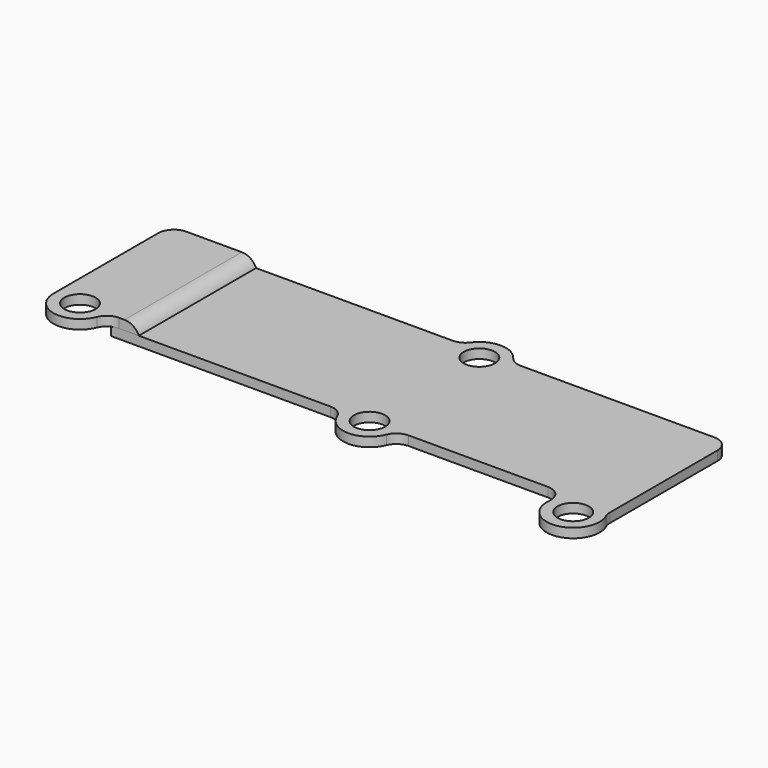
from build123d import *

# Parameters (mm, degrees)
F0_R          = 5
F1_DEPTH      = 3
F2_W          = 9
F2_H          = 47
F2_R          = 5
F3_DEPTH      = 3
F4_F1_R       = 5
F4_F2_R       = 5
F4_2_T1_DEPTH = 3
F4_2_T3_DEPTH = 69.9128784748
F4_2_T5_DEPTH = 28


# Not quite as in the source:
# - a fillet or chamfer that OpenCascade refuses, or shapes differently, is made with other operations: its cross-section is extruded or revolved along the edge and cut away or added


with BuildPart() as f1:
    # F0 (on Top) → F1 (new body)
    with BuildSketch(Plane.XY):
        with BuildLine():
            ThreePointArc((7.9529868603, 47), (0, 52.5), (-7.9529868603, 47))
            Line((-7.9529868603, 47), (-83, 47))
            Line((-83, 47), (-83, 0))
            Line((-83, 0), (-8.5, 0))
            ThreePointArc((-8.5, 0), (0, -8.5), (8.5, 0))
            Line((8.5, 0), (62.1807458666, 0))
            Line((62.1807458666, 0), (62.1807458666, -6.6735107167))
            Line((62.1807458666, -6.6735107167), (62.1807458666, -6.7810347379))
            ThreePointArc((62.1807458666, -6.7810347379), (72.9464615235, -14.9196937423), (78, -2.4056954659))
            Line((78, -2.4056954659), (78, 47))
            Line((78, 47), (7.9529868603, 47))
        make_face()
        Circle(F0_R, mode=Mode.SUBTRACT)
        with Locations((70.6805758441, -6.7272727273)):
            Circle(F0_R, mode=Mode.SUBTRACT)
        with Locations((0, 44)):
            Circle(F0_R, mode=Mode.SUBTRACT)
    extrude(amount=F1_DEPTH)

    # F4: fillet of radius 5 on 7 edges, made by hand

    # F4_f1
    f4_f1_edges = [f1.edges().sort_by_distance(p)[0] for p in [
        (8.5, 0, 1.5),
        (-8.5, 0, 1.5),
        (62.1807458666, 0, 1.5),
        (78, -2.4056954659, 1.5),
        (7.9529868603, 47, 1.5),
        (-7.9529868603, 47, 1.5),
    ]]
    fillet(f4_f1_edges, radius=F4_F1_R)

    # F4_f2
    f4_f2_edges = [f1.edges().sort_by_distance(p)[0] for p in [
        (78, 47, 1.5),
    ]]
    fillet(f4_f2_edges, radius=F4_F2_R)


with BuildPart() as f3:
    # F2 (on face) → F3 (new body)
    with BuildSketch(Plane.XY.offset(3)):
        with Locations((-78.5, 23.5)):
            Rectangle(F2_W, F2_H)
        with BuildLine():
            Line((-84.3662815094, 0), (-83, 0))
            Line((-83, 0), (-83, 47))
            Line((-83, 47), (-101.3662815094, 47))
            Line((-101.3662815094, 47), (-101.3662815094, 0))
            ThreePointArc((-101.3662815094, 0), (-92.8662815094, -8.5), (-84.3662815094, 0))
        make_face()
        with Locations((-92.8662815094, 0)):
            Circle(F2_R, mode=Mode.SUBTRACT)
    extrude(amount=F3_DEPTH)

    # F4#2: fillet of radius 5 on 3 edges, made by hand

    # F4_2_s2 → F4_2_t1 (join)
    with BuildSketch(Plane.XY.offset(3)):
        with BuildLine():
            ThreePointArc((-84.9707661217, -3.1481481481), (-83.1317633438, -0.8612043262), (-80.3263453054, 0))
            Line((-80.3263453054, 0), (-84.3662815094, 0))
            ThreePointArc((-84.3662815094, 0), (-84.5187704793, -1.6028286254), (-84.9707661217, -3.1481481481))
        make_face()
    extrude(amount=F4_2_T1_DEPTH)

    # F4_2_s4 → F4_2_t3 (cut)
    with BuildSketch(Plane.XZ.offset(-58.4564392374)):
        with BuildLine():
            ThreePointArc((-74, 3), (-75.8439629074, 5.1833001327), (-78.582575695, 6))
            Line((-78.582575695, 6), (-74, 6))
            Line((-74, 6), (-74, 3))
        make_face()
    extrude(amount=F4_2_T3_DEPTH, mode=Mode.SUBTRACT)

    # F4_2_s6 → F4_2_t5 (cut)
    with BuildSketch(Plane.XY.offset(-9.5)):
        with BuildLine():
            ThreePointArc((-96.3662815094, 47), (-99.9018154153, 45.5355339059), (-101.3662815094, 42))
            Line((-101.3662815094, 42), (-101.3662815094, 47))
            Line((-101.3662815094, 47), (-96.3662815094, 47))
        make_face()
    extrude(amount=F4_2_T5_DEPTH, mode=Mode.SUBTRACT)


solid = Compound([f1.part, f3.part])
